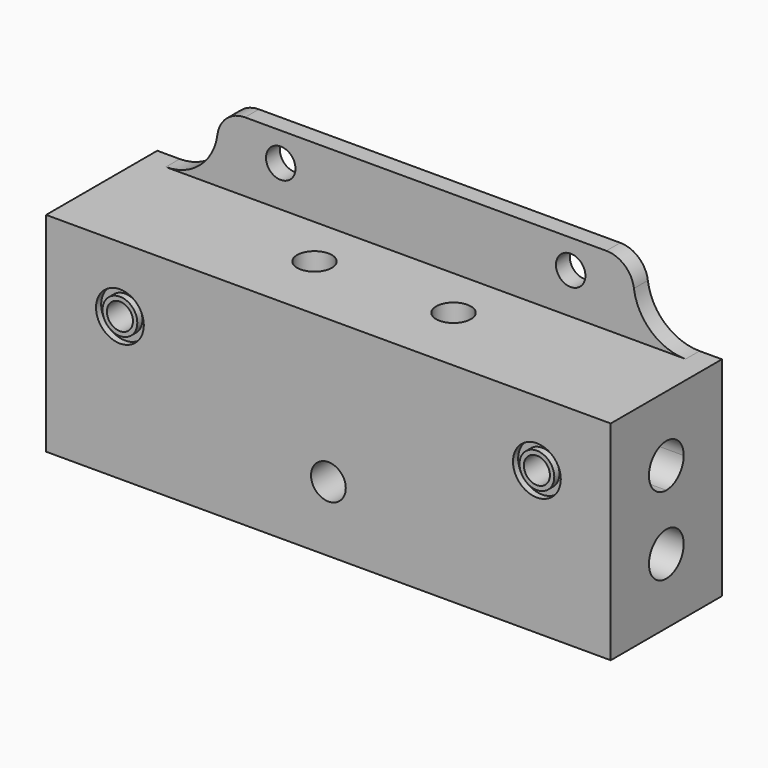
from build123d import *

# Parameters (mm, degrees)
F0_W         = 206.375
F0_H         = 76.2
F1_DEPTH     = 50.8
F2_R         = 6.35
F2_R_2       = 4.7625
F3_DEPTH     = 25.4
F5_DEPTH     = 206.376
F7_DEPTH     = 88.9
F9_DEPTH     = 88.9
F10_W        = 152.4
F10_H        = 127
F11_DEPTH    = 6.35
F12_R        = 10.16
F13_T1_DEPTH = 6.35
F14_R        = 5.3848
F15_DEPTH    = 25.4
F16_R        = 6.5786
F17_DEPTH    = 25.4
F18_R        = 6.35
F19_DEPTH    = 25.4
F20_R        = 6.35
F21_DEPTH    = 25.4
F22_R        = 9.6012
F23_DEPTH    = 2.286
F24_R        = 8.7376
F24_R_2      = 6.35
F25_DEPTH    = 2.3622


# Not quite as in the source:
# - a fillet or chamfer that OpenCascade refuses, or shapes differently, is made with other operations: its cross-section is extruded or revolved along the edge and cut away or added


with BuildPart() as f1:
    # F0 (on Front) → F1 (new body)
    with BuildSketch(Plane.XZ):
        Rectangle(F0_W, F0_H)
    extrude(amount=-F1_DEPTH)

    # F2 (on face) → F3 (cut)
    with BuildSketch(Plane.XZ):
        with Locations((0, -14.224)):
            Circle(F2_R)
        with Locations((-76.2, 14.224)):
            Circle(F2_R_2)
        with Locations((76.2, 14.224)):
            Circle(F2_R_2)
    extrude(amount=-F3_DEPTH, mode=Mode.SUBTRACT)

    # F4 (on face) → F5 (cut, through all)
    with BuildSketch(Plane(origin=(-103.1875, 0, 0), x_dir=(0, -1, 0), z_dir=(-1, 0, 0))):
        with BuildLine():
            ThreePointArc((-25.4, -6.2865), (-31.0126600757, -19.8366600757), (-17.4625, -14.224))
            Line((-17.4625, -14.224), (-25.4, -14.224))
            Line((-25.4, -14.224), (-25.4, -6.2865))
        make_face()
        with BuildLine():
            Line((-25.4, -14.224), (-17.4625, -14.224))
            ThreePointArc((-17.4625, -14.224), (-19.7873399243, -8.6113399243), (-25.4, -6.2865))
            Line((-25.4, -6.2865), (-25.4, -14.224))
        make_face()
    extrude(amount=-F5_DEPTH, mode=Mode.SUBTRACT)

    # F6 (on face) → F7 (cut)
    with BuildSketch(Plane(origin=(-103.1875, 0, 0), x_dir=(0, -1, 0), z_dir=(-1, 0, 0))):
        with BuildLine():
            ThreePointArc((-25.4, 6.2865), (-19.7873399243, 8.6113399243), (-17.4625, 14.224))
            ThreePointArc((-17.4625, 14.224), (-31.0126600757, 19.8366600757), (-25.4, 6.2865))
        make_face()
    extrude(amount=-F7_DEPTH, mode=Mode.SUBTRACT)

    # F8 (on face) → F9 (cut)
    with BuildSketch(Plane.YZ.offset(103.1875)):
        with BuildLine():
            ThreePointArc((25.4, 6.2865), (31.0126600757, 8.6113399243), (33.3375, 14.224))
            ThreePointArc((33.3375, 14.224), (19.7873399243, 19.8366600757), (25.4, 6.2865))
        make_face()
    extrude(amount=-F9_DEPTH, mode=Mode.SUBTRACT)

    # F10 (on face) → F11 (join)
    with BuildSketch(Plane(origin=(0, 50.8, 0), x_dir=(-1, 0, 0), z_dir=(0, 1, 0))):
        Rectangle(F10_W, F10_H)
    extrude(amount=-F11_DEPTH)

    # F12
    f12_edges = [f1.edges().sort_by_distance(p)[0] for p in [
        (-76.2, 47.625, 63.5),
        (76.2, 47.625, 63.5),
        (76.2, 47.625, -63.5),
        (-76.2, 47.625, -63.5),
    ]]
    fillet(f12_edges, radius=F12_R)

    # F13: fillet of radius 19.05 on 4 edges, made by hand

    # F13_s2 → F13_t1 (join)
    with BuildSketch(Plane.XZ.offset(-50.8)):
        with BuildLine():
            ThreePointArc((-76.1132020165, -54.6652173913), (-82.4392577793, -42.8280307099), (-95.0004557975, -38.1))
            Line((-95.0004557975, -38.1), (-95.0004557975, -36.195))
            Line((-95.0004557975, -36.195), (-76.2, -36.195))
            Line((-76.2, -36.195), (-74.295, -38.1))
            ThreePointArc((-74.295, -38.1), (-74.295, -53.34), (-74.2244766384, -54.4167391304))
            Line((-74.2244766384, -54.4167391304), (-76.1132020165, -54.6652173913))
        make_face()
        with BuildLine():
            ThreePointArc((95.0004557975, -38.1), (82.4392577793, -42.8280307099), (76.1132020165, -54.6652173913))
            Line((76.1132020165, -54.6652173913), (74.2244766384, -54.4167391304))
            ThreePointArc((74.2244766384, -54.4167391304), (74.295, -53.34), (74.295, -38.1))
            Line((74.295, -38.1), (76.2, -36.195))
            Line((76.2, -36.195), (95.0004557975, -36.195))
            Line((95.0004557975, -36.195), (95.0004557975, -38.1))
        make_face()
        with BuildLine():
            ThreePointArc((95.0004557975, 38.1), (82.4392577793, 42.8280307099), (76.1132020165, 54.6652173913))
            Line((76.1132020165, 54.6652173913), (74.2244766384, 54.4167391304))
            ThreePointArc((74.2244766384, 54.4167391304), (74.295, 53.34), (74.295, 38.1))
            Line((74.295, 38.1), (76.2, 36.195))
            Line((76.2, 36.195), (95.0004557975, 36.195))
            Line((95.0004557975, 36.195), (95.0004557975, 38.1))
        make_face()
        with BuildLine():
            ThreePointArc((-95.0004557975, 38.1), (-82.4392577793, 42.8280307099), (-76.1132020165, 54.6652173913))
            Line((-76.1132020165, 54.6652173913), (-74.2244766384, 54.4167391304))
            ThreePointArc((-74.2244766384, 54.4167391304), (-74.295, 53.34), (-74.295, 38.1))
            Line((-74.295, 38.1), (-76.2, 36.195))
            Line((-76.2, 36.195), (-95.0004557975, 36.195))
            Line((-95.0004557975, 36.195), (-95.0004557975, 38.1))
        make_face()
    extrude(amount=F13_T1_DEPTH)

    # F14 (on face) → F15 (cut)
    with BuildSketch(Plane(origin=(0, 50.8, 0), x_dir=(-1, 0, 0), z_dir=(0, 1, 0))):
        with Locations((-52.9844, 52.9844)):
            Circle(F14_R)
        with Locations((52.9844, 52.9844)):
            Circle(F14_R)
        with Locations((-52.9844, -52.9844)):
            Circle(F14_R)
        with Locations((52.9844, -52.9844)):
            Circle(F14_R)
    extrude(amount=-F15_DEPTH, mode=Mode.SUBTRACT)

    # F16 (on face) → F17 (cut)
    with BuildSketch(Plane(origin=(0, 50.8, 0), x_dir=(-1, 0, 0), z_dir=(0, 1, 0))):
        with Locations((-69.85, 14.224)):
            Circle(F16_R)
        with Locations((69.85, 14.224)):
            Circle(F16_R)
        with Locations((69.85, -14.224)):
            Circle(F16_R)
        with Locations((-69.85, -14.224)):
            Circle(F16_R)
    extrude(amount=-F17_DEPTH, mode=Mode.SUBTRACT)

    # F18 (on face) → F19 (cut)
    with BuildSketch(Plane.XY.offset(38.1)):
        with Locations((25.4, 25.4)):
            Circle(F18_R)
        with Locations((-25.4, 25.4)):
            Circle(F18_R)
    extrude(amount=-F19_DEPTH, mode=Mode.SUBTRACT)

    # F20 (on face) → F21 (cut)
    with BuildSketch(Plane(origin=(0, 0, -38.1), x_dir=(1, 0, 0), z_dir=(0, 0, -1))):
        with Locations((0, -25.4)):
            Circle(F20_R)
    extrude(amount=-F21_DEPTH, mode=Mode.SUBTRACT)

    # F22 (on face) → F23 (cut)
    with BuildSketch(Plane(origin=(0, 50.8, 0), x_dir=(-1, 0, 0), z_dir=(0, 1, 0))):
        with Locations((-69.85, 14.224)):
            Circle(F22_R)
        with Locations((-69.85, -14.224)):
            Circle(F22_R)
        with Locations((69.85, 14.224)):
            Circle(F22_R)
        with Locations((69.85, -14.224)):
            Circle(F22_R)
    extrude(amount=-F23_DEPTH, mode=Mode.SUBTRACT)

    # F24 (on face) → F25 (cut)
    with BuildSketch(Plane.XZ):
        with Locations((76.2, 14.224)):
            Circle(F24_R)
        with Locations((76.2, 14.224)):
            Circle(F24_R_2, mode=Mode.SUBTRACT)
        with Locations((-76.2, 14.224)):
            Circle(F24_R)
        with Locations((-76.2, 14.224)):
            Circle(F24_R_2, mode=Mode.SUBTRACT)
    extrude(amount=-F25_DEPTH, mode=Mode.SUBTRACT)


solid = f1.part
